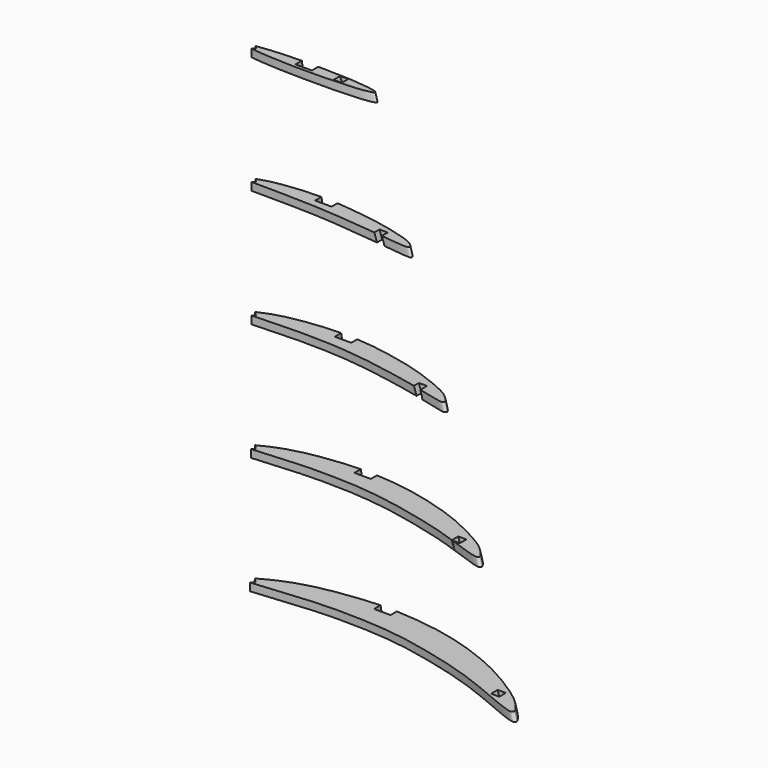
from build123d import *

# Parameters (mm, degrees)
F7_W           = 6.35
F7_H           = 3.175
F8_W           = 6.35
F8_H           = 3.175
F6_W           = 166.3111299276
F6_H           = 42.5
F10_DEPTH      = 25
F10_DEPTH_BACK = 25
F12_W          = 3.175
F12_H          = 3.175
F11_W          = 3.175
F11_H          = 3.175


with BuildPart() as f5:
    # F4 (on offset) → F5 section 0
    with BuildSketch(Plane.XY.offset(185)):
        with BuildLine():
            add(Edge.make_bspline(
                [(0, 0), (-0.0083768075, 0.1198584807), (0.4059524582, 0.3876821995), (0.7416993028, 0.6697443007), (3.0902344169, 1.1024557236), (5.2372779912, 1.4410683283), (9.0315599913, 1.813045489), (12.6054446403, 2.0598872326), (15.4294600639, 2.1702175429), (20.7319293167, 2.2968747383), (23.4226648099, 2.3370425722), (26.6994206566, 2.3511484567), (34.6620944874, 2.2003445627), (40.7563649369, 1.8718508202), (46.3604847627, 1.2409394934), (49.0675872721, 0.7126157973), (49.6464629837, 0.3750561458), (49.9153771702, 0.2032461413), (50.0345822795, 0.0044831733), (49.948475939, -0.1172067511), (49.8802514248, -0.1846088851), (49.6595739375, -0.3198063698), (49.3312019759, -0.5262402483), (46.2729837111, -1.2850658897), (41.1014839222, -1.6629846095), (33.3876358647, -2.0872460456), (28.6764588729, -2.1654137318), (21.7272115356, -2.1439414955), (20.8043254001, -2.1541153969), (12.8210491822, -1.9745365857), (9.1460017826, -1.651232028), (5.2930032674, -1.3784625491), (2.7029449392, -1.0189944434), (0.8543908151, -0.620399909), (0.4484846612, -0.3923817228), (0.3156290663, -0.2695258572), (0.0074956905, -0.1072511303), (0, 0)],
                knots=[0, 0, 0, 0, 0.013378751, 0.0265985732, 0.0547433457, 0.0839586697, 0.1209294221, 0.1567023374, 0.1893251646, 0.2327514051, 0.2638645276, 0.2976508222, 0.3510727565, 0.3996397793, 0.444862306, 0.4753997292, 0.4899320959, 0.5003799615, 0.5088653302, 0.5155503803, 0.5215058816, 0.5306056757, 0.5417179993, 0.5734467616, 0.6184288211, 0.6705699991, 0.7146572606, 0.7624396944, 0.7831811854, 0.835228905, 0.8744550186, 0.9107256342, 0.9422905963, 0.9677400463, 0.9796275931, 0.9880284969, 1, 1, 1, 1], degree=3))
        make_face()
    # F1 (on Top) → F5 section 1
    with BuildSketch(Plane.XY):
        with BuildLine():
            add(Edge.make_bspline(
                [(0, 0), (-0.0041649341, 0.0530320481), (0.0020486944, 0.1723425081), (0.1233394402, 0.5808732538), (1.7633052605, 1.726135133), (10.7199466748, 6.6217091948), (23.2115752666, 9.9237776706), (36.3980370302, 11.6151292651), (46.9163735359, 12.3102706761), (64.8374623071, 10.8221190269), (79.261750666, 7.140949741), (91.68182974, 2.4862337215), (101.4517630648, -2.7339434351), (108.0574717758, -6.9811551672), (115.2454260243, -12.0532052297), (119.1832195127, -17.3830423337), (118.5634760409, -17.7748271467), (117.9850224154, -18.7917194597), (109.4205343099, -15.3553561668), (96.6809930751, -9.7739612579), (83.5154287517, -5.406694744), (65.9552692874, -1.1697430017), (52.79465163, 0.7745065672), (36.6315166058, 1.3870508343), (24.9967233787, 0.982630733), (12.001912565, -0.388223704), (1.9681753065, -1.3423028894), (0.6566072994, -1.2096602836), (0.1134296621, -0.4148334001), (0.0294370081, -0.1832017302), (0.0042885102, -0.0546055413), (0, 0)],
                knots=[0, 0, 0, 0, 0.0052874359, 0.0127702719, 0.0295276725, 0.0707508132, 0.119480932, 0.1667415504, 0.2096793225, 0.2649648165, 0.3163834078, 0.3641681734, 0.4074857381, 0.4442327982, 0.4846972212, 0.515791928, 0.5238529014, 0.534508389, 0.5715433988, 0.6222121074, 0.6717109426, 0.7270126298, 0.7757925109, 0.8279303588, 0.8730975724, 0.9219079539, 0.9624351949, 0.9760738609, 0.988023305, 0.9945556826, 1, 1, 1, 1], degree=3))
        make_face()
    loft()

    # F7 (on Top) → F9 section 0
    with BuildSketch(Plane.XY):
        with Locations((46.1974537849, 10.4149581358)):
            Rectangle(F7_W, F7_H)
    # F8 (on offset) → F9 section 1
    with BuildSketch(Plane.XY.offset(185)):
        with Locations((22.962799567, 0.7943401046)):
            Rectangle(F8_W, F8_H)
    loft(mode=Mode.SUBTRACT)

    # F6 (on Front) → F10 (cut, two sides)
    with BuildSketch(Plane.XZ) as f10_sk:
        with Locations((60.1555649191, 24.25)):
            Rectangle(F6_W, F6_H)
        with Locations((60.1555649191, 69.75)):
            Rectangle(F6_W, F6_H)
        with Locations((60.1555649191, 115.25)):
            Rectangle(F6_W, F6_H)
        with Locations((60.1555649191, 160.75)):
            Rectangle(F6_W, F6_H)
    extrude(amount=-F10_DEPTH, mode=Mode.SUBTRACT)
    extrude(f10_sk.sketch, amount=F10_DEPTH_BACK, mode=Mode.SUBTRACT)

    # F12 (on Top) → F13 section 0
    with BuildSketch(Plane.XY):
        with Locations((107.6237160206, -11.1233041197)):
            Rectangle(F12_W, F12_H)
    # F11 (on offset) → F13 section 1
    with BuildSketch(Plane.XY.offset(185)):
        with Locations((36.6613428533, 0.1321118517)):
            Rectangle(F11_W, F11_H)
    loft(mode=Mode.SUBTRACT)

    # F14 (on face) → F16 section 0
    with BuildSketch(Plane(origin=(0, 0, 0), x_dir=(1, 0, 0), z_dir=(0, 0, -1))):
        Polygon((3.733523871, 0), (1.4884598407, 2.2450640303), (-0.7566041895, 0), (1.4884598407, -2.2450640303), align=None)
    # F15 (on face) → F16 section 1
    with BuildSketch(Plane.XY.offset(185)):
        Polygon((3.9631081745, 0), (1.7180441442, 2.2450640303), (-0.527019886, 0), (1.7180441442, -2.2450640303), align=None)
    loft(mode=Mode.SUBTRACT)


solid = f5.part
